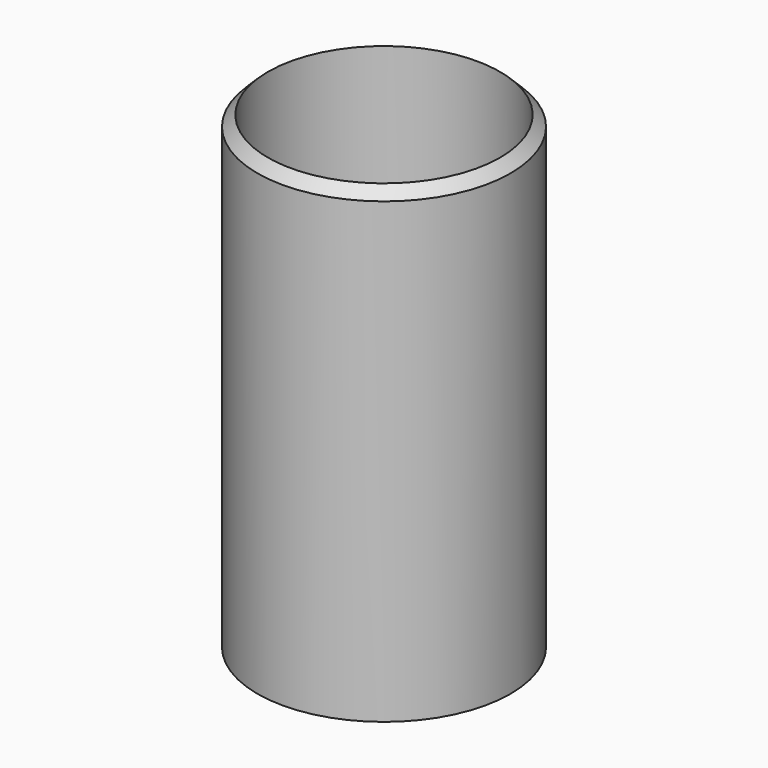
from build123d import *

# Parameters (mm, degrees)
F0_W     = 16.1361260527
F0_H     = 63.5
F2_R     = 14.8058887609
F3_DEPTH = 38.1


# Not quite as in the source:
# - a fillet or chamfer that OpenCascade refuses, or shapes differently, is made with other operations: its cross-section is extruded or revolved along the edge and cut away or added


with BuildPart() as f1:
    # F0 (on Front) → F1 (revolve)
    with BuildSketch(Plane.XZ):
        with Locations((-22.7458069295, 2.539942234)):
            Rectangle(F0_W, F0_H)
    revolve(axis=Axis((-14.6777439032, 0, 2.539942234), (0, 0, -1)))

    # F2 (on face) → F3 (cut)
    with BuildSketch(Plane.XY.offset(34.289942234)):
        with Locations((-14.6777439032, 0)):
            Circle(F2_R)
    extrude(amount=-F3_DEPTH, mode=Mode.SUBTRACT)

    # F4: chamfer of 5.08 on 1 edges, made by hand

    # F4_s1 → F4_t2 (revolve, cut)
    with BuildSketch(Plane.XZ):
        Polygon((-30.8138699559, 29.209942234), (-25.7338699559, 34.289942234), (-30.8138699559, 34.289942234), align=None)
    revolve(axis=Axis((-14.6777439032, 0, 34.289942234), (0, 0, -1)), mode=Mode.SUBTRACT)


solid = f1.part
